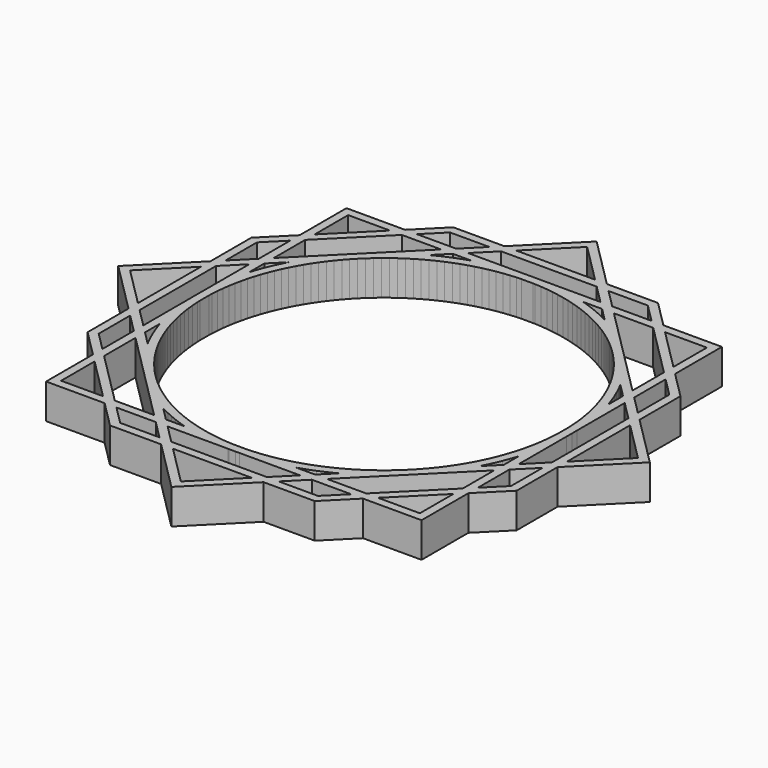
from build123d import *

# Parameters (mm, degrees)
F1_DEPTH = 3


with BuildPart() as f1:
    # F0 (on Top) → F1 (new body)
    with BuildSketch(Plane.XY):
        Polygon((15.4199172418, 0.5354985454), (15.4292124814, 0), (15.4199172418, -0.5354976467), (15.4197312112, -0.5390671289), (15.4197312112, -4.7881361488), (15.5294686006, -4.4270863431), (15.6737618498, -3.8854415981), (15.7991707454, -3.3391146333), (15.9055416099, -2.7887650936), (15.9927477268, -2.2350553199), (16.0606848472, -1.6786521464), (16.109269392, -1.1202260025), (16.1384429458, -0.5604509119), (16.1386900879, -0.5462131289), (16.1386900879, 0.5462131289), (16.1384429458, 0.5604509119), (16.1092684933, 1.1202269012), (16.0606839485, 1.6786521464), (15.9927468281, 2.2350553199), (15.9055407112, 2.7887650936), (15.799168948, 3.3391146333), (15.6737600524, 3.8854415981), (15.5294668032, 4.4270863431), (15.4197312112, 4.7881302351), (15.4197312112, 0.5390679065), align=None)
        Polygon((15.4199172418, -0.5354976467), (15.4292124814, 0), (15.4199172418, 0.5354985454), (15.4197312112, 0.5390679065), (15.4197312112, -0.5390671289), align=None)
        Polygon((15.4197312112, -4.7881361488), (15.4197312112, -0.5390671289), (15.3920423074, -1.0703509265), (15.3456209302, -1.6039136751), (15.2807088293, -2.1355451204), (15.1973850902, -2.6646017943), (15.0957503673, -3.1904492154), (14.9759250861, -3.7124511053), (14.8380557345, -4.229981071), (14.6823076731, -4.7424136182), (14.5088687297, -5.2491322398), (14.3179474026, -5.7495258206), (14.1097737585, -6.2429913339), (13.8845994331, -6.7289347401), (13.6426958333, -7.2067700874), (13.3843523402, -7.675922209), (13.1098825994, -8.1358258233), (12.8196164333, -8.5859255346), (12.5139043346, -9.0256803263), (12.193112972, -9.4545599664), (11.8576296849, -9.872047703), (11.5078597861, -10.2776402651), (11.144222968, -10.6708487605), (10.7671586942, -11.0512004738), (10.3771208075, -11.4182352712), (9.9745793272, -11.7715127906), (9.5600186518, -12.11060615), (9.1339393566, -12.4351082391), (8.6968545984, -12.7446254277), (8.2492901158, -13.0387874521), (7.7917869255, -13.3172384277), (7.3248941322, -13.5796431399), (6.8491761187, -13.8256852467), (6.365205356, -14.0550681776), (5.8735642008, -14.2675169309), (5.3748466928, -14.46277358), (4.8696531628, -14.6406044634), (4.358591131, -14.8007938933), (3.8422780032, -14.9431495483), (3.3213347803, -15.067499777), (2.7963896525, -15.1736953953), (2.2680753037, -15.2616078893), (1.7370280124, -15.331130314), (1.2038885509, -15.3821808877), (0.6692976911, -15.4146967016), (0.4759816107, -15.4197312112), (4.7873670304, -15.4197312112), (5.0965646726, -15.3228146559), (5.6252996124, -15.1366986702), (6.1472565673, -14.9323426977), (6.6618055497, -14.7099956781), (7.168328255, -14.4699236261), (7.5691270148, -14.2626293647), (14.2652170179, -7.5665396373), (14.2784073605, -7.5425858931), (14.5315833367, -7.0424843893), (14.7672508669, -6.5338973734), (14.985124165, -6.017436859), (15.1849417095, -5.4937265431), (15.3664626493, -4.9633964134), align=None)
        Polygon((15.3920414087, 1.0703509265), (15.4197312112, 0.5390679065), (15.4197312112, 4.7881302351), (15.3664608519, 4.9633964134), (15.1849390134, 5.4937265431), (14.9851214689, 6.017436859), (14.7672472722, 6.5338964747), (14.5315806406, 7.0424834906), (14.2784037657, 7.5425849944), (14.2652079164, 7.5665487387), (7.5691415627, 14.2626148169), (7.1683219641, 14.4699191326), (6.6617992588, 14.7099911846), (6.1472493777, 14.9323382042), (5.6252924228, 15.136693278), (5.096557483, 15.3228101624), (4.7873449855, 15.4197312112), (0.4756719228, 15.4197312112), (0.6692887041, 15.4146895121), (1.2038795639, 15.3821736982), (1.7370199241, 15.3311231244), (2.2680672154, 15.2616006997), (2.7963815642, 15.1736882057), (3.321326692, 15.0674934861), (3.8422699149, 14.9431432574), (4.3585830427, 14.8007876025), (4.8696450745, 14.6405981725), (5.3748386046, 14.4627681878), (5.8735570112, 14.2675115387), (6.3651972677, 14.0550636841), (6.8491689291, 13.8256807532), (7.3248869426, 13.5796386464), (7.7917797359, 13.3172339342), (8.2492829262, 13.0387838573), (8.6968474088, 12.7446218329), (9.133932167, 12.4351046443), (9.5600123609, 12.1106034539), (9.9745721376, 11.7715100945), (10.3771145166, 11.4182334738), (10.7671524033, 11.0511977777), (11.1442175758, 10.6708469631), (11.5078534952, 10.2776384677), (11.8576242927, 9.8720459057), (12.1931075798, 9.4545590677), (12.5138989424, 9.0256794276), (12.8196119399, 8.5859246359), (13.1098781059, 8.1358249246), (13.3843487454, 7.6759213103), (13.6426913399, 7.2067700874), (13.8845958383, 6.7289338414), (14.1097710624, 6.2429904352), (14.3179447065, 5.7495249219), (14.5088660336, 5.2491313411), (14.682304977, 4.7424136182), (14.8380539371, 4.229981071), (14.9759232887, 3.7124511053), (15.0957485699, 3.1904492154), (15.1973841915, 2.6646017943), (15.2807079306, 2.1355451204), (15.3456200315, 1.6039145738), align=None)
        Polygon((15.5294686006, -4.4270863431), (15.4197312112, -4.7881361488), (15.4197312112, -6.4120254915), (16.1386900879, -5.6930666443), (16.1386900879, -0.5462131289), (16.1384429458, -0.5604509119), (16.109269392, -1.1202260025), (16.0606848472, -1.6786521464), (15.9927477268, -2.2350553199), (15.9055416099, -2.7887650936), (15.7991707454, -3.3391146333), (15.6737618498, -3.8854415981), align=None)
        Polygon((15.4197312112, 6.4120254915), (15.4197312112, 4.7881302351), (15.5294668032, 4.4270863431), (15.6737600524, 3.8854415981), (15.799168948, 3.3391146333), (15.9055407112, 2.7887650936), (15.9927468281, 2.2350553199), (16.0606839485, 1.6786521464), (16.1092684933, 1.1202269012), (16.1384429458, 0.5604509119), (16.1386900879, 0.5462131289), (16.1386900879, 5.6930666443), align=None)
        Polygon((16.1386900879, -5.6930666443), (15.4197312112, -6.4120254915), (15.4197312112, -7.4287869925), (16.1386900879, -6.709828144), align=None)
        Polygon((15.4197312112, -7.4287869925), (15.4197312112, -6.4120254915), (14.2652170179, -7.5665396373), (14.0080266983, -8.033598858), (13.7207675778, -8.514932839), (13.4169750992, -8.9860063781), (13.0970168303, -9.4462523966), (12.7612783127, -9.8951163973), (12.4101621634, -10.3320573638), (12.044093467, -10.7565495573), (11.6635125855, -11.1680807196), (11.2688787542, -11.5661556679), (10.860665587, -11.9502935984), (10.4393664696, -12.3200325799), (10.0054891667, -12.6749268581), (9.5595558221, -13.0145486523), (9.1021038575, -13.3384899534), (8.6336841754, -13.6463580301), (8.1548620569, -13.937784416), (7.666213568, -14.2124159226), (7.5691270148, -14.2626293647), (6.4120251207, -15.4197312112), (7.4287866782, -15.4197312112), align=None)
        Polygon((14.2652079164, 7.5665487387), (15.4197312112, 6.4120254915), (15.4197312112, 7.4287869925), (7.4287866782, 15.4197312112), (6.4120251207, 15.4197312112), (7.5691415627, 14.2626148169), (7.6662072771, 14.2124123278), (8.154855766, 13.9377808212), (8.6336778845, 13.646355334), (9.1020975666, 13.3384863586), (9.5595495312, 13.0145459562), (10.0054828758, 12.674924162), (10.4393610774, 12.3200298839), (10.8606601948, 11.9502909023), (11.2688724633, 11.5661529718), (11.6635071933, 11.1680789223), (12.0440889735, 10.7565477599), (12.4101576699, 10.3320564651), (12.7612729205, 9.8951145999), (13.0970123368, 9.4462505992), (13.4169715044, 8.9860045807), (13.7207630843, 8.5149310416), (14.0080231035, 8.0335979593), align=None)
        Polygon((15.4197312112, 7.4287869925), (15.4197312112, 6.4120254915), (16.1386900879, 5.6930666443), (16.1386900879, 6.709828144), align=None)
        Polygon((16.1386900879, -6.709828144), (15.4197312112, -7.4287869925), (15.4197312112, -10.8066760443), (16.1386900879, -10.0877172376), align=None)
        Polygon((17.7240060943, -4.1077507032), (16.1386900879, -5.6930666443), (16.1386900879, -6.709828144), (17.7240060943, -5.1245122), align=None)
        Polygon((14.0080266983, -8.033598858), (14.2652170179, -7.5665396373), (7.5691270148, -14.2626293647), (7.666213568, -14.2124159226), (8.1548620569, -13.937784416), (8.6336841754, -13.6463580301), (9.1021038575, -13.3384899534), (9.5595558221, -13.0145486523), (10.0054891667, -12.6749268581), (10.4393664696, -12.3200325799), (10.860665587, -11.9502935984), (11.2688787542, -11.5661556679), (11.6635125855, -11.1680807196), (12.044093467, -10.7565495573), (12.4101621634, -10.3320573638), (12.7612783127, -9.8951163973), (13.0970168303, -9.4462523966), (13.4169750992, -8.9860063781), (13.7207675778, -8.514932839), align=None)
        Polygon((15.4197312112, 10.8066760443), (15.4197312112, 7.4287869925), (16.1386900879, 6.709828144), (16.1386900879, 10.0877172376), align=None)
        Polygon((7.5691415627, 14.2626148169), (14.2652079164, 7.5665487387), (14.0080231035, 8.0335979593), (13.7207630843, 8.5149310416), (13.4169715044, 8.9860045807), (13.0970123368, 9.4462505992), (12.7612729205, 9.8951145999), (12.4101576699, 10.3320564651), (12.0440889735, 10.7565477599), (11.6635071933, 11.1680789223), (11.2688724633, 11.5661529718), (10.8606601948, 11.9502909023), (10.4393610774, 12.3200298839), (10.0054828758, 12.674924162), (9.5595495312, 13.0145459562), (9.1020975666, 13.3384863586), (8.6336778845, 13.646355334), (8.154855766, 13.9377808212), (7.6662072771, 14.2124123278), align=None)
        Polygon((16.1386900879, 6.709828144), (16.1386900879, 5.6930666443), (17.7240060943, 4.1077507032), (17.7240060943, 5.1245122), align=None)
        Polygon((16.1386900879, -10.0877172376), (15.4197312112, -10.8066760443), (15.4197312112, -11.8234372346), (16.1386900879, -11.1044784918), align=None)
        Polygon((15.4197312112, -11.8234372346), (15.4197312112, -10.8066760443), (10.8066755947, -15.4197312112), (11.8234365642, -15.4197312112), align=None)
        Polygon((6.7098277731, -16.1386900879), (7.4287866782, -15.4197312112), (6.4120251207, -15.4197312112), (5.6930662143, -16.1386900879), align=None)
        Polygon((10.8066755947, -15.4197312112), (7.4287866782, -15.4197312112), (6.7098277731, -16.1386900879), (10.0877166479, -16.1386900879), align=None)
        Polygon((16.1386900879, 0.5462131289), (16.1386900879, -0.5462131289), (16.1481713581, 0), align=None)
        Polygon((18.4429649711, -3.3887918561), (17.7240060943, -4.1077507032), (17.7240060943, -5.1245122), (18.4429649711, -4.4055533515), align=None)
        Polygon((17.7240060943, 4.1077507032), (17.7240060943, -4.1077507032), (18.4429649711, -3.3887918561), (18.4429649711, 3.3887918561), align=None)
        Polygon((10.8066755947, 15.4197312112), (15.4197312112, 10.8066760443), (15.4197312112, 11.8234372346), (11.8234365642, 15.4197312112), align=None)
        Polygon((15.4197312112, 11.8234372346), (15.4197312112, 10.8066760443), (16.1386900879, 10.0877172376), (16.1386900879, 11.1044784918), align=None)
        Polygon((6.7098277731, 16.1386900879), (7.4287866782, 15.4197312112), (10.8066755947, 15.4197312112), (10.0877166479, 16.1386900879), align=None)
        Polygon((6.4120251207, 15.4197312112), (7.4287866782, 15.4197312112), (6.7098277731, 16.1386900879), (5.6930662143, 16.1386900879), align=None)
        Polygon((17.7240060943, 5.1245122), (17.7240060943, 4.1077507032), (18.4429649711, 3.3887918561), (18.4429649711, 4.4055533515), align=None)
        Polygon((16.1386900879, -11.1044784918), (15.4197312112, -11.8234372346), (15.4197312112, -15.4197312112), (11.8234365642, -15.4197312112), (11.1044775534, -16.1386900879), (16.1386900879, -16.1386900879), align=None)
        Polygon((11.8234365642, -15.4197312112), (10.8066755947, -15.4197312112), (10.0877166479, -16.1386900879), (11.1044775534, -16.1386900879), align=None)
        Polygon((17.7240060943, -8.5024013858), (16.1386900879, -10.0877172376), (16.1386900879, -11.1044784918), (18.4429649711, -8.8002040382), (18.4429649711, -4.4055533515), (17.7240060943, -5.1245122), align=None)
        Polygon((5.6930662143, -16.1386900879), (6.4120251207, -15.4197312112), (4.7873670304, -15.4197312112), (4.561689824, -15.4904686764), (4.0213176362, -15.6394585244), (3.4760996655, -15.7696026629), (2.9266937593, -15.8807465156), (2.3737613599, -15.9727552779), (1.8179693015, -16.0455184097), (1.2599862159, -16.0989469399), (0.7004852284, -16.1329788584), (0.4811714801, -16.1386900879), align=None)
        Polygon((5.1245117044, -17.7240060943), (6.7098277731, -16.1386900879), (5.6930662143, -16.1386900879), (4.1077501427, -17.7240060943), align=None)
        Polygon((21.8317569666, 0), (18.4429649711, -3.3887918561), (18.4429649711, -4.4055533515), (22.8485184958, 0), (18.4429649711, 4.4055533515), (18.4429649711, 3.3887918561), align=None)
        Polygon((15.4197312112, 15.4197312112), (15.4197312112, 11.8234372346), (16.1386900879, 11.1044784918), (16.1386900879, 16.1386900879), (11.1044775534, 16.1386900879), (11.8234365642, 15.4197312112), align=None)
        Polygon((16.1386900879, 11.1044784918), (16.1386900879, 10.0877172376), (17.7240060943, 8.5024013858), (17.7240060943, 5.1245122), (18.4429649711, 4.4055533515), (18.4429649711, 8.8002040382), align=None)
        Polygon((10.0877166479, 16.1386900879), (10.8066755947, 15.4197312112), (11.8234365642, 15.4197312112), (11.1044775534, 16.1386900879), align=None)
        Polygon((4.7873449855, 15.4197312112), (6.4120251207, 15.4197312112), (5.6930662143, 16.1386900879), (0.4808741358, 16.1386900879), (0.7004771401, 16.1329716688), (1.2599781276, 16.098940649), (1.8179612132, 16.0455112201), (2.3737541703, 15.972748987), (2.9266865697, 15.8807411234), (3.4760924759, 15.7695972707), (4.0213095479, 15.6394522335), (4.5616817358, 15.4904641829), align=None)
        Polygon((5.6930662143, 16.1386900879), (6.7098277731, 16.1386900879), (5.1245117044, 17.7240060943), (4.1077501427, 17.7240060943), align=None)
        Polygon((11.1044775534, -16.1386900879), (10.0877166479, -16.1386900879), (8.5024004871, -17.7240060943), (5.1245117044, -17.7240060943), (4.4055527994, -18.4429649711), (8.8002022408, -18.4429649711), align=None)
        Polygon((4.561689824, -15.4904686764), (4.7873670304, -15.4197312112), (0.4759816107, -15.4197312112), (0.1338997999, -15.4286400104), (-0.4016580596, -15.4239919412), (-0.4997893427, -15.4197312112), (-4.7932968477, -15.4197312112), (-4.2921494451, -15.5673101024), (-3.7492725842, -15.7068986644), (-3.2018788642, -15.827560634), (-2.6506261324, -15.9291513207), (-2.0961803245, -16.0115494002), (-1.5392082749, -16.0746551169), (-0.98038221, -16.1183911828), (-0.5128741753, -16.1386900879), (0.4811714801, -16.1386900879), (0.7004852284, -16.1329788584), (1.2599862159, -16.0989469399), (1.8179693015, -16.0455184097), (2.3737613599, -15.9727552779), (2.9266937593, -15.8807465156), (3.4760996655, -15.7696026629), (4.0213176362, -15.6394585244), align=None)
        Polygon((4.4055527994, -18.4429649711), (5.1245117044, -17.7240060943), (4.1077501427, -17.7240060943), (3.3887912364, -18.4429649711), align=None)
        Polygon((8.5024004871, 17.7240060943), (10.0877166479, 16.1386900879), (11.1044775534, 16.1386900879), (8.8002022408, 18.4429649711), (4.4055527994, 18.4429649711), (5.1245117044, 17.7240060943), align=None)
        Polygon((0.4756719228, 15.4197312112), (4.7873449855, 15.4197312112), (4.5616817358, 15.4904641829), (4.0213095479, 15.6394522335), (3.4760924759, 15.7695972707), (2.9266865697, 15.8807411234), (2.3737541703, 15.972748987), (1.8179612132, 16.0455112201), (1.2599781276, 16.098940649), (0.7004771401, 16.1329716688), (0.4808741358, 16.1386900879), (-0.5126959807, 16.1386900879), (-0.9803902983, 16.1183830945), (-1.5392163632, 16.0746461299), (-2.0961884128, 16.0115413119), (-2.6506342207, 15.9291432324), (-3.2018860538, 15.827551647), (-3.7492806725, 15.7068887787), (-4.2921566346, 15.5673011154), (-4.7932706752, 15.4197312112), (-0.4995911809, 15.4197312112), (-0.4016670466, 15.4239829542), (0.1338917116, 15.4286310234), align=None)
        Polygon((4.1077501427, 17.7240060943), (5.1245117044, 17.7240060943), (4.4055527994, 18.4429649711), (3.3887912364, 18.4429649711), align=None)
        Polygon((0.1338997999, -15.4286400104), (0.4759816107, -15.4197312112), (-0.4997893427, -15.4197312112), (-0.4016580596, -15.4239919412), align=None)
        Polygon((0.1401394643, -16.1475710275), (0.4811714801, -16.1386900879), (-0.5128741753, -16.1386900879), (-0.4203743565, -16.142706372), align=None)
        Polygon((3.3887912364, -18.4429649711), (4.1077501427, -17.7240060943), (-4.1077499736, -17.7240060943), (-3.3887910969, -18.4429649711), align=None)
        Polygon((0, -22.8485175971), (4.4055527994, -18.4429649711), (3.3887912364, -18.4429649711), (0, -21.8317560679), (-3.3887910969, -18.4429649711), (-4.4055526261, -18.4429649711), align=None)
        Polygon((-0.4995911809, 15.4197312112), (0.4756719228, 15.4197312112), (0.1338917116, 15.4286310234), (-0.4016670466, 15.4239829542), align=None)
        Polygon((-0.5126959807, 16.1386900879), (0.4808741358, 16.1386900879), (0.1401322747, 16.1475629392), (-0.4203824448, 16.1426982837), align=None)
        Polygon((-4.1077499736, 17.7240060943), (4.1077501427, 17.7240060943), (3.3887912364, 18.4429649711), (-3.3887910969, 18.4429649711), align=None)
        Polygon((3.3887912364, 18.4429649711), (4.4055527994, 18.4429649711), (0, 22.8485175971), (-4.4055526261, 18.4429649711), (-3.3887910969, 18.4429649711), (0, 21.8317560679), align=None)
        Polygon((-4.7932968477, -15.4197312112), (-0.4997893427, -15.4197312112), (-0.9367333179, -15.4007596838), (-1.4706789122, -15.3589701991), (-2.0028531714, -15.2986747129), (-2.5326135263, -15.2199451211), (-3.0593227994, -15.1228775844), (-3.5823456109, -15.0075871364), (-4.101051973, -14.8742139738), (-4.6148163915, -14.7229189639), (-5.1230214606, -14.5538836437), (-5.6250524703, -14.3673120178), (-6.1203063938, -14.1634296595), (-6.6081855967, -13.9424810149), (-7.0881032287, -13.7047320987), (-7.5594796293, -13.4504704946), (-8.0217468209, -13.1800026586), (-8.4743494078, -12.8936530211), (-8.9167409812, -12.5917684796), (-9.3483877143, -12.2747112098), (-9.7687710578, -11.9428640571), (-10.1773841458, -11.5966269425), (-10.5737335928, -11.2364159635), (-10.9573430885, -10.8626669888), (-11.3277498031, -10.4758284691), (-11.6845070834, -10.0763686262), (-12.0271853516, -9.6647664667), (-12.3553721048, -9.2415189707), (-12.6686710172, -8.8071365992), (-12.9667064325, -8.3621423946), (-13.2491170741, -7.9070719813), (-13.5155632339, -7.4424744643), (-13.765724975, -6.9689097326), (-13.9992994362, -6.4869475613), (-14.2160062235, -5.9971694083), (-14.4155838155, -5.5001648199), (-14.5977922597, -4.996533228), (-14.7624104763, -4.4868812542), (-14.9092416503, -3.9718227097), (-15.0381087381, -3.4519785952), (-15.1488553661, -2.9279753035), (-15.2413494256, -2.4004437212), (-15.3154785792, -1.8700192281), (-15.371153856, -1.3373425963), (-15.4083078533, -0.8030536992), (-15.4197303125, -0.4741471798), (-15.4197303125, -4.7905916123), (-15.27800824, -5.2293563771), (-15.0873097901, -5.7564565842), (-14.878432465, -6.2766197367), (-14.6516279004, -6.7892203406), (-14.4071693005, -7.2936400911), (-14.2605383562, -7.5712177118), (-7.5704379748, -14.2613180931), (-7.4183884432, -14.3433338405), (-6.9161093927, -14.5921610143), (-6.4054958115, -14.82340515), (-5.8871642067, -15.0367885498), (-5.3617400725, -15.2320532873), (-4.8298542955, -15.4089657007), align=None)
        Polygon((-5.69306598, -16.1386900879), (-0.5128741753, -16.1386900879), (-0.98038221, -16.1183911828), (-1.5392082749, -16.0746551169), (-2.0961803245, -16.0115494002), (-2.6506261324, -15.9291513207), (-3.2018788642, -15.827560634), (-3.7492725842, -15.7068986644), (-4.2921494451, -15.5673101024), (-4.7932968477, -15.4197312112), (-6.4120248568, -15.4197312112), align=None)
        Polygon((-3.3887910969, -18.4429649711), (-4.1077499736, -17.7240060943), (-5.1245115028, -17.7240060943), (-4.4055526261, -18.4429649711), align=None)
        Polygon((-5.1245115028, -17.7240060943), (-4.1077499736, -17.7240060943), (-5.69306598, -16.1386900879), (-6.7098275092, -16.1386900879), align=None)
        Polygon((-0.9367414062, 15.4007506968), (-0.4995911809, 15.4197312112), (-4.7932706752, 15.4197312112), (-4.8298614851, 15.408955815), (-5.3617472621, 15.2320434016), (-5.8871713962, 15.0367777655), (-6.405503001, 14.8233943656), (-6.9161156836, 14.5921502299), (-7.4183956328, 14.3433230562), (-7.5704538948, 14.2613021732), (-14.2605303176, 7.5712257504), (-14.4071728953, 7.2936266106), (-14.6516305965, 6.7892059614), (-14.8784351611, 6.2766053575), (-15.0873124862, 5.7564413063), (-15.2780109361, 5.229341998), (-15.4197303125, 4.7905825522), (-15.4197303125, 0.4741404277), (-15.408308752, 0.8030375226), (-15.3711547547, 1.337325521), (-15.3154794779, 1.8700030515), (-15.2413503243, 2.4004266459), (-15.1488571635, 2.9279582282), (-15.0381105355, 3.4519624186), (-14.9092443464, 3.9718065331), (-14.7624131724, 4.4868650776), (-14.5977949558, 4.9965170514), (-14.4155874103, 5.5001486433), (-14.2160098183, 5.9971532317), (-13.999303031, 6.4869322834), (-13.7657285698, 6.9688944548), (-13.5155677274, 7.4424591864), (-13.2491206689, 7.9070567035), (-12.966710926, 8.3621271167), (-12.6686764094, 8.8071213213), (-12.3553765983, 9.2415045915), (-12.0271907438, 9.6647511888), (-11.6845124756, 10.0763533484), (-11.3277551953, 10.4758140899), (-10.9573484807, 10.8626526096), (-10.5737398837, 11.236402483), (-10.1773904367, 11.5966125634), (-9.7687782474, 11.9428505766), (-9.3483949039, 12.2746977293), (-8.9167472721, 12.5917549991), (-8.4743565974, 12.8936404393), (-8.0217540105, 13.1799900768), (-7.5594868189, 13.4504588115), (-7.0881104183, 13.7047204156), (-6.608193685, 13.9424684331), (-6.1203144821, 14.1634179764), (-5.6250605585, 14.3673012334), (-5.1230295489, 14.5538728593), (-4.6148244798, 14.7229081795), (-4.1010600613, 14.8742040882), (-3.5823536992, 15.0075772507), (-3.0593308877, 15.1228676988), (-2.5326216146, 15.2199361341), (-2.0028612597, 15.2986648272), (-1.4706878991, 15.3589612121), align=None)
        Polygon((-0.9803902983, 16.1183830945), (-0.5126959807, 16.1386900879), (-5.69306598, 16.1386900879), (-6.4120248568, 15.4197312112), (-4.7932706752, 15.4197312112), (-4.2921566346, 15.5673011154), (-3.7492806725, 15.7068887787), (-3.2018860538, 15.827551647), (-2.6506342207, 15.9291432324), (-2.0961884128, 16.0115413119), (-1.5392163632, 16.0746461299), align=None)
        Polygon((-5.69306598, 16.1386900879), (-4.1077499736, 17.7240060943), (-5.1245115028, 17.7240060943), (-6.7098275092, 16.1386900879), align=None)
        Polygon((-5.1245115028, 17.7240060943), (-4.1077499736, 17.7240060943), (-3.3887910969, 18.4429649711), (-4.4055526261, 18.4429649711), align=None)
        Polygon((-6.7098275092, -16.1386900879), (-5.69306598, -16.1386900879), (-6.4120248568, -15.4197312112), (-7.428786386, -15.4197312112), align=None)
        Polygon((-4.4055526261, -18.4429649711), (-5.1245115028, -17.7240060943), (-8.5023915001, -17.7240060943), (-10.0877090514, -16.1386900879), (-11.1044711832, -16.1386900879), (-8.8001941525, -18.4429649711), align=None)
        Polygon((-6.4120248568, 15.4197312112), (-5.69306598, 16.1386900879), (-6.7098275092, 16.1386900879), (-7.428786386, 15.4197312112), align=None)
        Polygon((-8.5023915001, 17.7240060943), (-5.1245115028, 17.7240060943), (-4.4055526261, 18.4429649711), (-8.8001941525, 18.4429649711), (-11.1044711832, 16.1386900879), (-10.0877090514, 16.1386900879), align=None)
        Polygon((-7.428786386, -15.4197312112), (-6.4120248568, -15.4197312112), (-7.5704379748, -14.2613180931), (-7.9117299362, -14.0772246928), (-8.3955380344, -13.794152609), (-8.8692303813, -13.4944608921), (-9.3322363031, -13.1785090215), (-9.7839968094, -12.8466780455), (-10.2239690862, -12.4993669861), (-10.6516220027, -12.1369964343), (-11.0664397058, -11.7600013603), (-11.4679243166, -11.3688356068), (-11.8555905377, -10.9639718893), (-12.2289719447, -10.5458982012), (-12.5876182895, -10.1151169149), (-12.9310972981, -9.6721474783), (-13.2589955691, -9.2175237182), (-13.5709185739, -8.7517938409), (-13.866488859, -8.2755186343), (-14.1453505398, -7.7892723668), (-14.2605383562, -7.5712177118), (-15.4197303125, -6.4120257555), (-15.4197303125, -7.4287872847), align=None)
        Polygon((-10.0877090514, -16.1386900879), (-6.7098275092, -16.1386900879), (-7.428786386, -15.4197312112), (-10.8066686288, -15.4197312112), align=None)
        Polygon((-7.5704538948, 14.2613021732), (-6.4120248568, 15.4197312112), (-7.428786386, 15.4197312112), (-15.4197303125, 7.4287872847), (-15.4197303125, 6.4120257555), (-14.2605303176, 7.5712257504), (-14.1453541346, 7.7892579876), (-13.8664924538, 8.2755051538), (-13.5709221687, 8.7517803604), (-13.2590000626, 9.2175102377), (-12.9311017916, 9.6721339978), (-12.587622783, 10.1151034344), (-12.2289773369, 10.5458847207), (-11.8555959299, 10.9639593075), (-11.4679297088, 11.368823025), (-11.0664459967, 11.7599878798), (-10.6516273949, 12.1369838525), (-10.2239744784, 12.499355303), (-9.7840031003, 12.8466654637), (-9.332242594, 13.1784964398), (-8.8692366721, 13.4944492091), (-8.3955443253, 13.7941418246), (-7.9117362271, 14.0772130097), align=None)
        Polygon((-7.428786386, 15.4197312112), (-6.7098275092, 16.1386900879), (-10.0877090514, 16.1386900879), (-10.8066686288, 15.4197312112), align=None)
        Polygon((-7.9117299362, -14.0772246928), (-7.5704379748, -14.2613180931), (-14.2605383562, -7.5712177118), (-14.1453505398, -7.7892723668), (-13.866488859, -8.2755186343), (-13.5709185739, -8.7517938409), (-13.2589955691, -9.2175237182), (-12.9310972981, -9.6721474783), (-12.5876182895, -10.1151169149), (-12.2289719447, -10.5458982012), (-11.8555905377, -10.9639718893), (-11.4679243166, -11.3688356068), (-11.0664397058, -11.7600013603), (-10.6516220027, -12.1369964343), (-10.2239690862, -12.4993669861), (-9.7839968094, -12.8466780455), (-9.3322363031, -13.1785090215), (-8.8692303813, -13.4944608921), (-8.3955380344, -13.794152609), align=None)
        Polygon((-11.1044711832, -16.1386900879), (-10.0877090514, -16.1386900879), (-10.8066686288, -15.4197312112), (-11.82343073, -15.4197312112), align=None)
        Polygon((-16.1386891892, -16.1386900879), (-11.1044711832, -16.1386900879), (-11.82343073, -15.4197312112), (-15.4197303125, -15.4197312112), (-15.4197303125, -11.8234349805), (-16.1386891892, -11.1044767737), align=None)
        Polygon((-14.2605303176, 7.5712257504), (-7.5704538948, 14.2613021732), (-7.9117362271, 14.0772130097), (-8.3955443253, 13.7941418246), (-8.8692366721, 13.4944492091), (-9.332242594, 13.1784964398), (-9.7840031003, 12.8466654637), (-10.2239744784, 12.499355303), (-10.6516273949, 12.1369838525), (-11.0664459967, 11.7599878798), (-11.4679297088, 11.368823025), (-11.8555959299, 10.9639593075), (-12.2289773369, 10.5458847207), (-12.587622783, 10.1151034344), (-12.9311017916, 9.6721339978), (-13.2590000626, 9.2175102377), (-13.5709221687, 8.7517803604), (-13.8664924538, 8.2755051538), (-14.1453541346, 7.7892579876), align=None)
        Polygon((-10.8066686288, 15.4197312112), (-10.0877090514, 16.1386900879), (-11.1044711832, 16.1386900879), (-11.82343073, 15.4197312112), align=None)
        Polygon((-11.82343073, 15.4197312112), (-11.1044711832, 16.1386900879), (-16.1386891892, 16.1386900879), (-16.1386891892, 11.1044767737), (-15.4197303125, 11.8234349805), (-15.4197303125, 15.4197312112), align=None)
        Polygon((-11.82343073, -15.4197312112), (-10.8066686288, -15.4197312112), (-15.4197303125, -10.8066740232), (-15.4197303125, -11.8234349805), align=None)
        Polygon((-16.1386891892, -6.7098284079), (-15.4197303125, -7.4287872847), (-15.4197303125, -6.4120257555), (-16.1386891892, -5.6930668787), align=None)
        Polygon((-15.4197303125, -10.8066740232), (-15.4197303125, -7.4287872847), (-16.1386891892, -6.7098284079), (-16.1386891892, -10.0877158471), align=None)
        Polygon((-15.4197303125, 10.8066740232), (-10.8066686288, 15.4197312112), (-11.82343073, 15.4197312112), (-15.4197303125, 11.8234349805), align=None)
        Polygon((-16.1386891892, 6.7098284079), (-15.4197303125, 7.4287872847), (-15.4197303125, 10.8066740232), (-16.1386891892, 10.0877158471), align=None)
        Polygon((-15.4197303125, 6.4120257555), (-15.4197303125, 7.4287872847), (-16.1386891892, 6.7098284079), (-16.1386891892, 5.6930668787), align=None)
        Polygon((-15.4197303125, -11.8234349805), (-15.4197303125, -10.8066740232), (-16.1386891892, -10.0877158471), (-16.1386891892, -11.1044767737), align=None)
        Polygon((-16.1386891892, -5.6930668787), (-15.4197303125, -6.4120257555), (-15.4197303125, -4.7905916123), (-15.4502977478, -4.695956293), (-15.6039707142, -4.1568971038), (-15.7388420073, -3.6128294673), (-15.8547498613, -3.0644094335), (-15.9515531806, -2.5122957484), (-16.0291369317, -1.9571561452), (-16.0874058526, -1.3996574582), (-16.1262916421, -0.8404728126), (-16.1386891892, -0.4834753432), align=None)
        Polygon((-17.7240051956, -5.1245124015), (-16.1386891892, -6.7098284079), (-16.1386891892, -5.6930668787), (-17.7240051956, -4.1077508723), align=None)
        Polygon((-18.4429640724, -8.8002040382), (-16.1386891892, -11.1044767737), (-16.1386891892, -10.0877158471), (-17.7240051956, -8.5024013858), (-17.7240051956, -5.1245124015), (-18.4429640724, -4.4055535248), align=None)
        Polygon((-16.1386891892, 10.0877158471), (-15.4197303125, 10.8066740232), (-15.4197303125, 11.8234349805), (-16.1386891892, 11.1044767737), align=None)
        Polygon((-15.4197303125, 4.7905825522), (-15.4197303125, 6.4120257555), (-16.1386891892, 5.6930668787), (-16.1386891892, 0.4834600653), (-16.1262916421, 0.8404575347), (-16.0874067513, 1.3996421803), (-16.0291378304, 1.9571408673), (-15.9515540793, 2.5122813692), (-15.85475076, 3.0643941556), (-15.7388438047, 3.6128150881), (-15.6039725116, 4.1568827246), (-15.4502995452, 4.6959410151), align=None)
        Polygon((-16.1386891892, 5.6930668787), (-16.1386891892, 6.7098284079), (-17.7240051956, 5.1245124015), (-17.7240051956, 4.1077508723), align=None)
        Polygon((-16.1386891892, 10.0877158471), (-16.1386891892, 11.1044767737), (-18.4429640724, 8.8002040382), (-18.4429640724, 4.4055535248), (-17.7240051956, 5.1245124015), (-17.7240051956, 8.5024013858), align=None)
        Polygon((-15.4502977478, -4.695956293), (-15.4197303125, -4.7905916123), (-15.4197303125, -0.4741471798), (-15.4268965351, -0.2677978024), (-15.4268965351, 0.2677807271), (-15.4197303125, 0.4741404277), (-15.4197303125, 4.7905825522), (-15.4502995452, 4.6959410151), (-15.6039725116, 4.1568827246), (-15.7388438047, 3.6128150881), (-15.85475076, 3.0643941556), (-15.9515540793, 2.5122813692), (-16.0291378304, 1.9571408673), (-16.0874067513, 1.3996421803), (-16.1262916421, 0.8404575347), (-16.1386891892, 0.4834600653), (-16.1386891892, -0.4834753432), (-16.1262916421, -0.8404728126), (-16.0874058526, -1.3996574582), (-16.0291369317, -1.9571561452), (-15.9515531806, -2.5122957484), (-15.8547498613, -3.0644094335), (-15.7388420073, -3.6128294673), (-15.6039707142, -4.1568971038), align=None)
        Polygon((-18.4429640724, -4.4055535248), (-17.7240051956, -5.1245124015), (-17.7240051956, -4.1077508723), (-18.4429640724, -3.3887919956), align=None)
        Polygon((-17.7240051956, 4.1077508723), (-17.7240051956, 5.1245124015), (-18.4429640724, 4.4055535248), (-18.4429640724, 3.3887919956), align=None)
        Polygon((-15.4268965351, -0.2677978024), (-15.4197303125, -0.4741471798), (-15.4197303125, 0.4741404277), (-15.4268965351, 0.2677807271), align=None)
        Polygon((-16.1457457706, -0.2802753337), (-16.1386891892, -0.4834753432), (-16.1386891892, 0.4834600653), (-16.1457457706, 0.2802600558), align=None)
        Polygon((-18.4429640724, -3.3887919956), (-17.7240051956, -4.1077508723), (-17.7240051956, 4.1077508723), (-18.4429640724, 3.3887919956), align=None)
        Polygon((-22.8485175971, 0), (-18.4429640724, -4.4055535248), (-18.4429640724, -3.3887919956), (-21.8317560679, 0), (-18.4429640724, 3.3887919956), (-18.4429640724, 4.4055535248), align=None)
    extrude(amount=F1_DEPTH)


solid = f1.part
